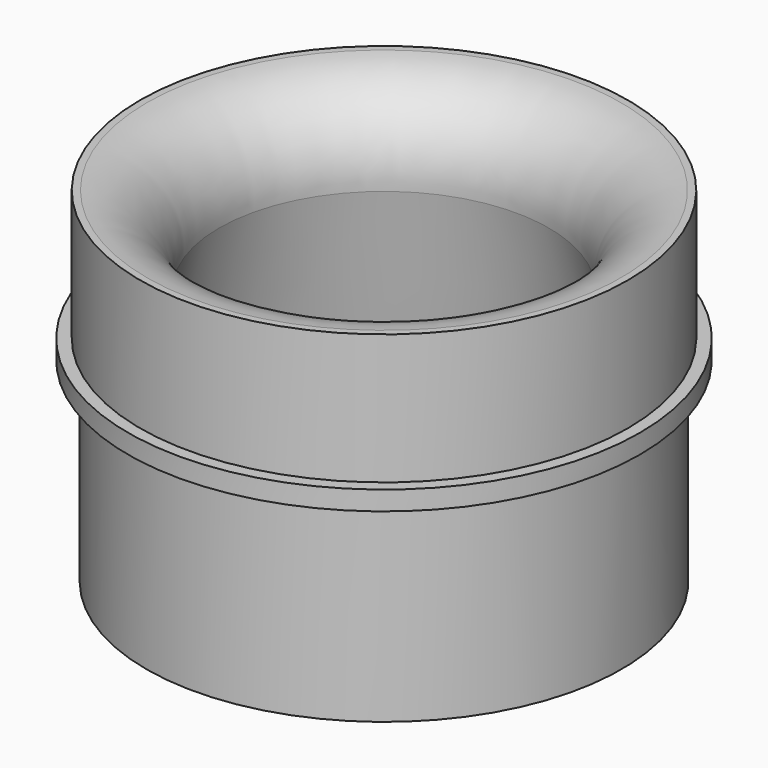
from build123d import *


# Not quite as in the source:
# - a feature names something its author has since deleted; it is built from what else it names


with BuildPart() as f1:
    # F0 (on Front) → F1 (revolve)
    with BuildSketch(Plane.XZ):
        with BuildLine():
            Line((-19.9644, 0.412851112), (-20.955, 0.412851112))
            Line((-20.955, 0.412851112), (-20.955, -1.161948888))
            Line((-20.955, -1.161948888), (-19.4564, -1.161948888))
            Line((-19.4564, -1.161948888), (-19.4564, -17.113148888))
            Line((-19.4564, -17.113148888), (-19.0119, -17.113148888))
            ThreePointArc((-19.0119, -17.113148888), (-17.0327575285, -13.4915583263), (-15.8800452648, -9.52870865))
            Line((-15.8800452648, -9.52870865), (-13.5, 3.9691987902))
            ThreePointArc((-13.5, 3.9691987902), (-14.9174256152, 8.8000179565), (-19.4056, 11.080851112))
            Line((-19.4056, 11.080851112), (-19.9644, 11.080851112))
            Line((-19.9644, 11.080851112), (-19.9644, 0.412851112))
        make_face()
    revolve(axis=Axis((0, 0, 12.5831294567), (0, 0, -1)))


solid = f1.part
